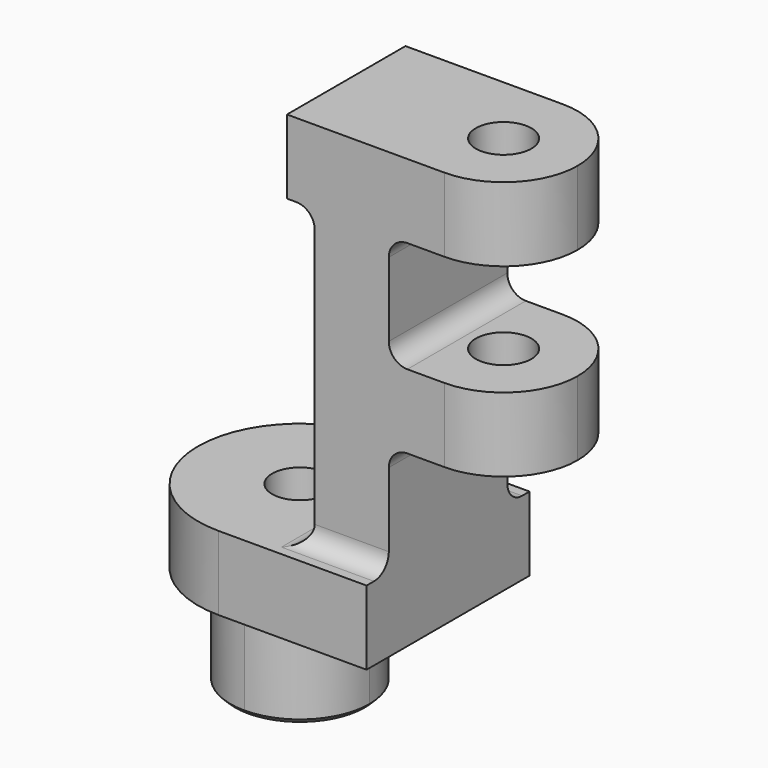
from build123d import *

# Parameters (mm, degrees)
F1_DEPTH  = 11
F2_W      = 8
F2_H      = 45
F2_W_2    = 8.5
F2_H_2    = 15
F3_DEPTH  = 25
F4_R      = 7.49999
F5_R      = 10.99999
F6_R      = 7.99999
F7_R      = 2
F8_R      = 3
F9_DEPTH  = 19
F10_R     = 3
F11_DEPTH = 35
F12_SIZE  = 0.5


# Not quite as in the source:
# - a fillet or chamfer is up to 0.001 mm smaller than in the source, because OpenCascade refuses the exact size


with BuildPart() as f1:
    # F0 (on Front) → F1 (new body, symmetric)
    with BuildSketch(Plane.XZ):
        Polygon((-15, -11), (0, -11), (0, 0), (8.5, 0), (8.5, 20), (22.5, 20), (22.5, 28), (8.5, 28), (8.5, 40), (22.5, 40), (22.5, 48), (-2.5, 48), (-2.5, 40), (0.5, 40), (0.5, 8), (-18.5, 8), (-18.5, 0), (-15, 0), align=None)
    extrude(amount=F1_DEPTH, both=True)

    # F2 (on Right) → F3 (cut, symmetric)
    with BuildSketch(Plane.YZ):
        with Locations((-12, 30.5)):
            Rectangle(F2_W, F2_H)
        with Locations((12, 30.5)):
            Rectangle(F2_W, F2_H)
        with Locations((-11.75, -7.5)):
            Rectangle(F2_W_2, F2_H_2)
        with Locations((11.75, -7.5)):
            Rectangle(F2_W_2, F2_H_2)
    extrude(amount=F3_DEPTH, both=True, mode=Mode.SUBTRACT)

    # F4 (radius 7.5 in the source; OpenCascade refuses exactly that, so slightly less here)
    f4_edges = [f1.edges().sort_by_distance(p)[0] for p in [
        (0, -7.5, -5.5),
        (-15, -7.5, -5.5),
        (0, 7.5, -5.5),
        (-15, 7.5, -5.5),
    ]]
    fillet(f4_edges, radius=F4_R)

    # F5 (radius 11 in the source; OpenCascade refuses exactly that, so slightly less here)
    f5_edges = [f1.edges().sort_by_distance(p)[0] for p in [
        (-18.5, 11, 4),
        (-18.5, -11, 4),
    ]]
    fillet(f5_edges, radius=F5_R)

    # F6 (radius 8 in the source; OpenCascade refuses exactly that, so slightly less here)
    f6_edges = [f1.edges().sort_by_distance(p)[0] for p in [
        (22.5, 8, 44),
        (22.5, 8, 24),
        (22.5, -8, 24),
        (22.5, -8, 44),
    ]]
    fillet(f6_edges, radius=F6_R)

    # F7
    f7_edges = [f1.edges().sort_by_distance(p)[0] for p in [
        (8.5, 0, 28),
        (8.5, 0, 40),
        (0.5, 0, 40),
        (0.5, 0, 8),
        (4.5, -8, 8),
        (4.5, 8, 8),
        (8.5, 0, 20),
    ]]
    fillet(f7_edges, radius=F7_R)

    # F8 (on face) → F9 (cut)
    with BuildSketch(Plane.XY.offset(8)):
        with Locations((-7.5, 0)):
            Circle(F8_R)
    extrude(amount=-F9_DEPTH, mode=Mode.SUBTRACT)

    # F10 (on face) → F11 (cut)
    with BuildSketch(Plane.XY.offset(48)):
        with Locations((14.5, 0)):
            Circle(F10_R)
    extrude(amount=-F11_DEPTH, mode=Mode.SUBTRACT)

    # F12
    f12_edges = [f1.edges().sort_by_distance(p)[0] for p in [
        (-12.803304, -5.303304, -11),
    ]]
    chamfer(f12_edges, length=F12_SIZE)


solid = f1.part
